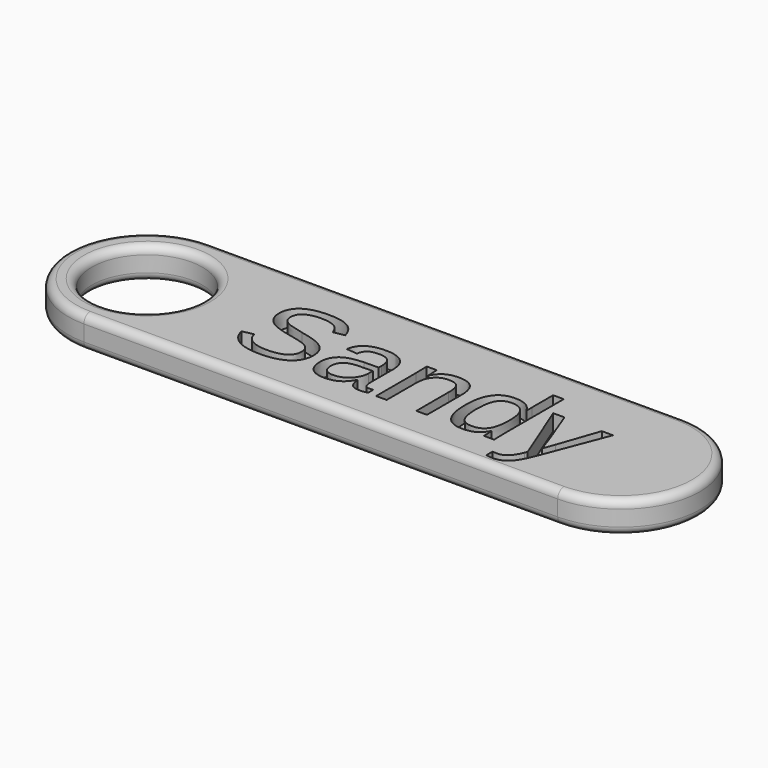
from build123d import *

# Parameters (mm, degrees)
F0_R         = 8.89
F1_DEPTH     = 5.08
F2_TEXT_SIZE = 19.4027777778
F3_DEPTH     = 2.54
F4_R         = 1.27


# Not quite as in the source:
# - Text() gives the source's letters only with a copy of the font that has no kerning and outlines rounded to 1/6400 em; it was checked with that copy


with BuildPart() as f1:
    # F0 (on Top) → F1 (new body)
    with BuildSketch(Plane.XY):
        with BuildLine():
            Line((-38.1, -12.7), (38.1, -12.7))
            ThreePointArc((38.1, -12.7), (50.8, 0), (38.1, 12.7))
            Line((38.1, 12.7), (-38.1, 12.7))
            ThreePointArc((-38.1, 12.7), (-50.8, 0), (-38.1, -12.7))
        make_face()
        with Locations((-38.1, 0)):
            Circle(F0_R, mode=Mode.SUBTRACT)
    extrude(amount=F1_DEPTH)

    # F2 (on face) → F3 (cut)
    with BuildSketch(Plane.XY.offset(5.08)):
        with Locations((-20.7626258681, -6.985)):
            Text('Sandy', F2_TEXT_SIZE, font='Arimo', text_align=(TextAlign.LEFT, TextAlign.BOTTOM))
    extrude(amount=-F3_DEPTH, mode=Mode.SUBTRACT)

    # F4
    f4_edges = [f1.edges().sort_by_distance(p)[0] for p in [
        (-50.8, 0, 5.08),
        (0, -12.7, 0),
        (50.8, 0, 0),
        (0, 12.7, 0),
        (-50.8, 0, 0),
        (-46.99, 0, 0),
        (-46.99, 0, 5.08),
    ]]
    fillet(f4_edges, radius=F4_R)


solid = f1.part
